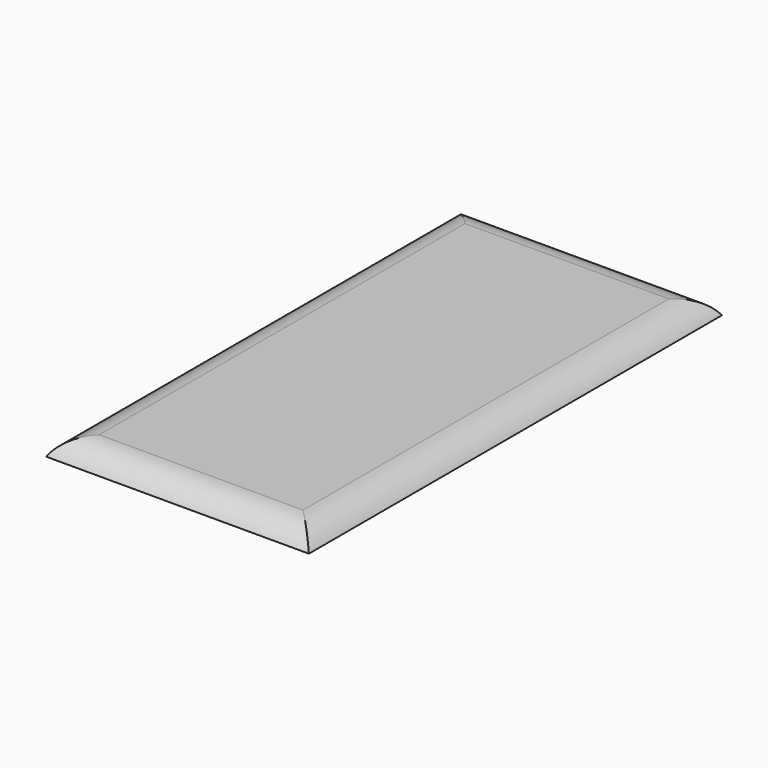
from build123d import *

# Parameters (mm, degrees)
F0_W        = 39.0131762251
F0_H        = 76.6465999186
F1_DEPTH    = 2.5021
F2_T1_DEPTH = 98.5331434957
F2_T3_DEPTH = 60.8997198022


# Not quite as in the source:
# - a fillet or chamfer that OpenCascade refuses, or shapes differently, is made with other operations: its cross-section is extruded or revolved along the edge and cut away or added


with BuildPart() as f1:
    # F0 (on Top) → F1 (new body)
    with BuildSketch(Plane.XY):
        with Locations((-30.2404207177, 3.7039015442)):
            Rectangle(F0_W, F0_H)
    extrude(amount=F1_DEPTH)

    # F2: fillet of radius 5.08 on 4 edges, made by hand

    # F2_s2 → F2_t1 (cut)
    with BuildSketch(Plane.XZ.offset(-52.970473292)):
        with BuildLine():
            ThreePointArc((-10.7338326052, 0), (-12.5901625424, 1.8324362684), (-15.1111413206, 2.5021))
            Line((-15.1111413206, 2.5021), (-10.7338326052, 2.5021))
            Line((-10.7338326052, 2.5021), (-10.7338326052, 0))
        make_face()
        with BuildLine():
            ThreePointArc((-49.7470088303, 0), (-47.8906788931, 1.8324362684), (-45.3697001149, 2.5021))
            Line((-45.3697001149, 2.5021), (-49.7470088303, 2.5021))
            Line((-49.7470088303, 2.5021), (-49.7470088303, 0))
        make_face()
    extrude(amount=F2_T1_DEPTH, mode=Mode.SUBTRACT)

    # F2_s4 → F2_t3 (cut)
    with BuildSketch(Plane.YZ.offset(-60.6902806188)):
        with BuildLine():
            ThreePointArc((-34.6193984151, 0), (-32.7630684779, 1.8324362684), (-30.2420896997, 2.5021))
            Line((-30.2420896997, 2.5021), (-34.6193984151, 2.5021))
            Line((-34.6193984151, 2.5021), (-34.6193984151, 0))
        make_face()
        with BuildLine():
            ThreePointArc((42.0272015035, 0), (40.1708715663, 1.8324362684), (37.6498927881, 2.5021))
            Line((37.6498927881, 2.5021), (42.0272015035, 2.5021))
            Line((42.0272015035, 2.5021), (42.0272015035, 0))
        make_face()
    extrude(amount=F2_T3_DEPTH, mode=Mode.SUBTRACT)


solid = f1.part
